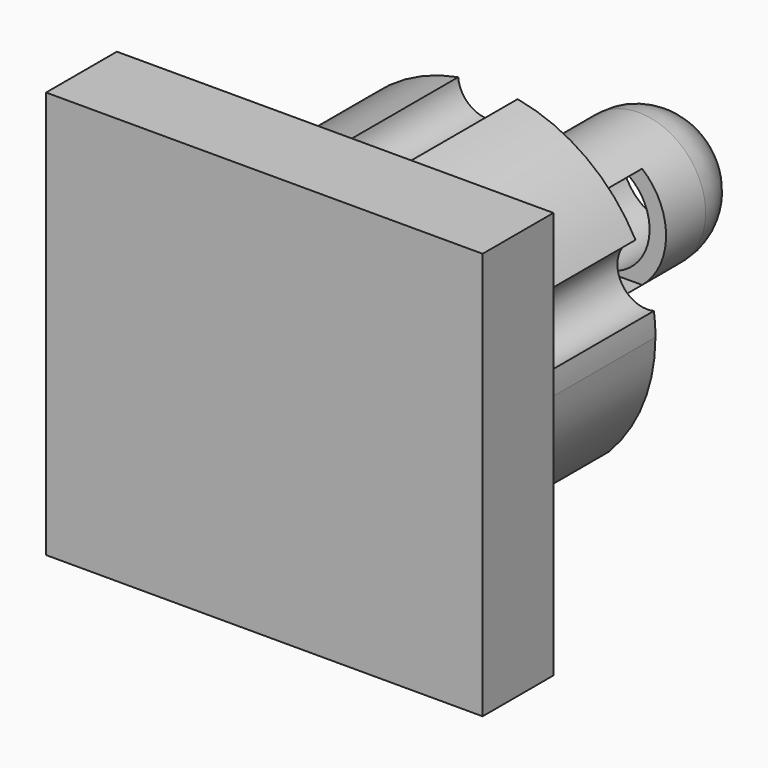
from build123d import *

# Parameters (mm, degrees)
F0_W          = 125.3066509962
F0_H          = 116.8914437294
F2_DEPTH      = 25.4
F3_DEPTH      = 54.8134744167
F4_R          = 19.141083189
F4_R_2        = 14.402572036
F5_DEPTH      = 65.8841822296
F7_W          = 17.8398638964
F7_H          = 29.3952524662
F8_DEPTH      = 25.4
F8_DEPTH_BACK = 25.4


# Not quite as in the source:
# - a fillet or chamfer that OpenCascade refuses, or shapes differently, is made with other operations: its cross-section is extruded or revolved along the edge and cut away or added


with BuildPart() as f2:
    # F0 (on Front) → F2 (new body)
    with BuildSketch(Plane.XZ):
        Rectangle(F0_W, F0_H)
    extrude(amount=F2_DEPTH)

    # F1 (on face) → F3 (join)
    with BuildSketch(Plane.XZ):
        with BuildLine():
            ThreePointArc((34.7187500455, -33.271908015), (44.6203470202, -17.9286390861), (48.0875396302, 0))
            ThreePointArc((48.0875396302, 0), (47.9767259565, 3.262703507), (47.6447956571, 6.5103697647))
            ThreePointArc((47.6447956571, 6.5103697647), (37.5878279083, 12.213025626), (42.3721487148, 22.7379084564))
            ThreePointArc((42.3721487148, 22.7379084564), (28.2651466136, 38.9036367785), (8.5313219634, 47.3247082742))
            ThreePointArc((8.5313219634, 47.3247082742), (0, 39.5221811368), (-8.5313219634, 47.3247082742))
            ThreePointArc((-8.5313219634, 47.3247082742), (-28.2651466136, 38.9036367785), (-42.3721487148, 22.7379084564))
            ThreePointArc((-42.3721487148, 22.7379084564), (-38.5869212276, 19.5805755678), (-37.1686094245, 14.8598669634))
            ThreePointArc((-37.1686094245, 14.8598669634), (-40.3955017751, 8.1616473967), (-47.6447956571, 6.5103697647))
            ThreePointArc((-47.6447956571, 6.5103697647), (-45.7339679179, -14.8598669634), (-34.7187500455, -33.271908015))
            ThreePointArc((-34.7187500455, -33.271908015), (-25.2578272797, -30.88357465), (-19.6997881202, -38.9036367785))
            ThreePointArc((-19.6997881202, -38.9036367785), (-20.0091221024, -41.1847385714), (-20.9147811398, -43.3010784803))
            ThreePointArc((-20.9147811398, -43.3010784803), (0, -48.0875396302), (20.9147811398, -43.3010784803))
            ThreePointArc((20.9147811398, -43.3010784803), (23.2305552106, -31.9741161944), (34.7187500455, -33.271908015))
        make_face()
    extrude(amount=-F3_DEPTH)

    # F4 (on face) → F5 (join)
    with BuildSketch(Plane(origin=(0, 54.8134744167, 0), x_dir=(-1, 0, 0), z_dir=(0, 1, 0))):
        Circle(F4_R)
        Circle(F4_R_2, mode=Mode.SUBTRACT)
    extrude(amount=F5_DEPTH)

    # F6: fillet of radius 16.8234648582 on 1 edges, made by hand

    # F6_s1 → F6_t2 (revolve, cut)
    with BuildSketch(Plane.XY):
        with BuildLine():
            ThreePointArc((-19.141083189, 108.9936887817), (-17.9115236115, 115.3070941964), (-14.402572036, 120.6976566464))
            Line((-14.402572036, 120.6976566464), (-19.141083189, 120.6976566464))
            Line((-19.141083189, 120.6976566464), (-19.141083189, 108.9936887817))
        make_face()
    revolve(axis=Axis((0, 120.6976566464, 0), (0, 1, 0)), mode=Mode.SUBTRACT)

    # F7 (on Right) → F8 (cut, two sides)
    with BuildSketch(Plane.YZ) as f8_sk:
        with Locations((85.9047025442, 0)):
            Rectangle(F7_W, F7_H)
    extrude(amount=-F8_DEPTH, mode=Mode.SUBTRACT)
    extrude(f8_sk.sketch, amount=F8_DEPTH_BACK, mode=Mode.SUBTRACT)


solid = f2.part
